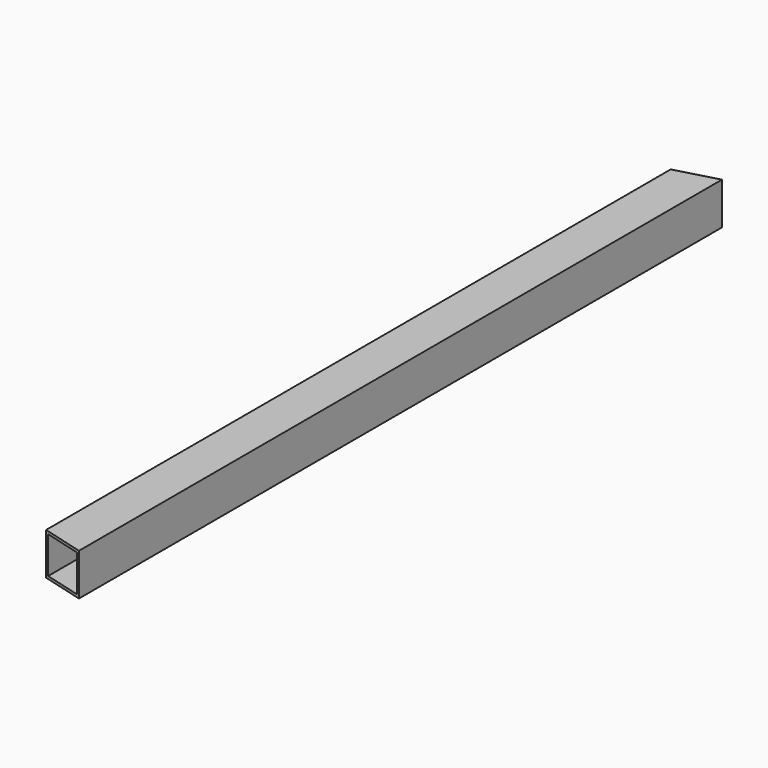
from build123d import *

# Parameters (mm, degrees)
F0_W     = 25.4
F0_H     = 25.4
F0_W_2   = 22.225
F0_H_2   = 22.225
F1_DEPTH = 242.57
F3_DEPTH = 25.401


# Not quite as in the source:
# - a pattern or mirror of a feature is missing from the dataset's text; its kind, count and spacing are read off the source's solid


with BuildPart() as f1:
    # F0 (on Front) → F1 (new body, symmetric)
    with BuildSketch(Plane.XZ):
        Rectangle(F0_W, F0_H)
        Rectangle(F0_W_2, F0_H_2, mode=Mode.SUBTRACT)
    extrude(amount=F1_DEPTH, both=True)

    # F2 (on face) → F3 (cut, through all)
    with BuildSketch(Plane.XY.offset(12.7)):
        Polygon((12.7, 242.57), (-12.7, 242.57), (-12.7, 235.6213463057), align=None)
    f3 = extrude(amount=-F3_DEPTH, mode=Mode.SUBTRACT)

    # F3_copies: F3 across plane
    add(f3.mirror(Plane(origin=(0, 0, 0), x_dir=(0, 0, -1), z_dir=(0, -1, 0))), mode=Mode.SUBTRACT)


solid = f1.part
